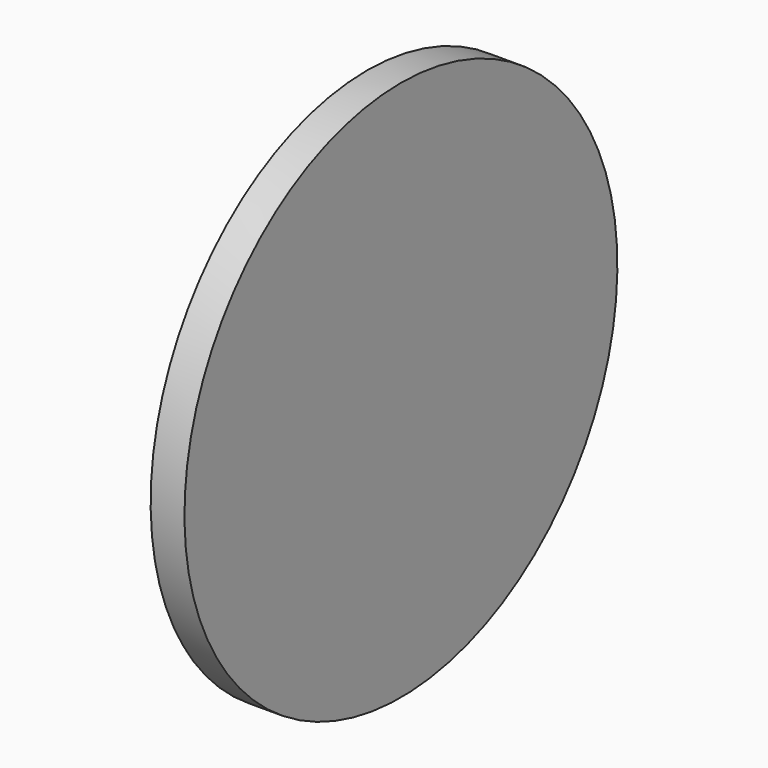
from build123d import *


# Not quite as in the source:
# - a feature of the source that left no trace in its solid (it failed there, or was rolled back) is left out


with BuildPart() as f1:
    # F0 (on Front) → F1 (revolve)
    with BuildSketch(Plane.XZ):
        with BuildLine():
            Line((-15.24, 0), (0, 0))
            Line((0, 0), (0, 50.8))
            Line((0, 50.8), (-6.35, 50.8))
            Line((-6.35, 50.8), (-4.7617064118, 41.792339449))
            ThreePointArc((-4.7617064118, 41.792339449), (-4.8311637627, 41.5331210865), (-5.0743828734, 41.4197061526))
            Line((-5.0743828734, 41.4197061526), (-6.2835011077, 41.4197061526))
            ThreePointArc((-6.2835011077, 41.4197061526), (-6.5080075107, 41.3267125556), (-6.6010011077, 41.1022061526))
            Line((-6.6010011077, 41.1022061526), (-6.6010011077, 40.4672061526))
            ThreePointArc((-6.6010011077, 40.4672061526), (-6.5080075107, 40.2426997495), (-6.2835011077, 40.1497061526))
            Line((-6.2835011077, 40.1497061526), (-5.0743828734, 40.1497061526))
            ThreePointArc((-5.0743828734, 40.1497061526), (-4.8311637627, 40.0362912186), (-4.7617064118, 39.7770728561))
            Line((-4.7617064118, 39.7770728561), (-5.2010717431, 37.2853082403))
            ThreePointArc((-5.2010717431, 37.2853082403), (-5.3096631386, 37.0972224261), (-5.5137482047, 37.0229415367))
            Line((-5.5137482047, 37.0229415367), (-6.8348340718, 37.0229415367))
            ThreePointArc((-6.8348340718, 37.0229415367), (-7.0593404748, 36.9299479398), (-7.1523340718, 36.7054415367))
            Line((-7.1523340718, 36.7054415367), (-7.1523340718, 36.0704415367))
            ThreePointArc((-7.1523340718, 36.0704415367), (-7.2453276688, 35.8459351337), (-7.4698340718, 35.7529415367))
            Line((-7.4698340718, 35.7529415367), (-8.7398340718, 35.7529415367))
            ThreePointArc((-8.7398340718, 35.7529415367), (-8.9643404748, 35.6599479398), (-9.0573340718, 35.4354415367))
            Line((-9.0573340718, 35.4354415367), (-9.0573340718, 34.8004415367))
            ThreePointArc((-9.0573340718, 34.8004415367), (-8.9643404748, 34.5759351337), (-8.7398340718, 34.4829415367))
            Line((-8.7398340718, 34.4829415367), (-3.5686493249, 34.4829415367))
            ThreePointArc((-3.5686493249, 34.4829415367), (-3.3254302142, 34.3695266028), (-3.2559728633, 34.1103082403))
            Line((-3.2559728633, 34.1103082403), (-7.113602572, 12.2326030065))
            ThreePointArc((-7.113602572, 12.2326030065), (-7.2221939675, 12.0445171922), (-7.4262790336, 11.9702363029))
            Line((-7.4262790336, 11.9702363029), (-8.1123649007, 11.9702363029))
            ThreePointArc((-8.1123649007, 11.9702363029), (-8.3368713037, 11.8772427059), (-8.4298649007, 11.6527363029))
            Line((-8.4298649007, 11.6527363029), (-8.4298649007, 8.9432889844))
            ThreePointArc((-8.4298649007, 8.9432889844), (-8.4596121783, 8.8091076862), (-8.5432798346, 8.7000698737))
            Line((-8.5432798346, 8.7000698737), (-15.1265850661, 3.176020882))
            ThreePointArc((-15.1265850661, 3.176020882), (-15.2102527224, 3.0669830694), (-15.24, 2.9328017713))
            Line((-15.24, 2.9328017713), (-15.24, 0))
        make_face()
    revolve(axis=Axis((-7.62, 0, 0), (-1, 0, 0)))


solid = f1.part
